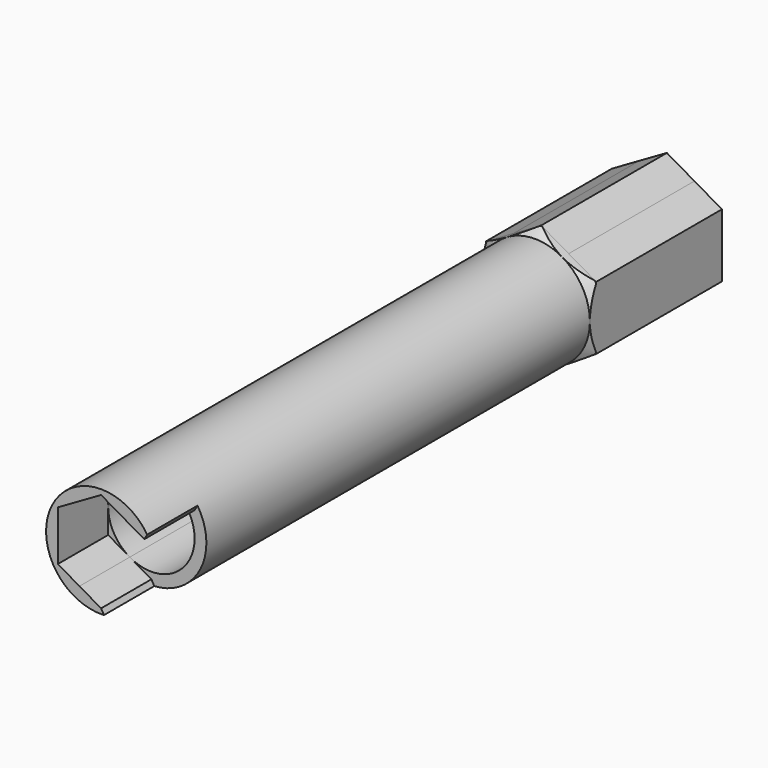
from build123d import *

# Parameters (mm, degrees)
F0_R         = 7
F1_DEPTH     = 70
F2_DEPTH     = 62
F3_R         = 5.5
F4_DEPTH     = 20
F6_DEPTH     = 8
F7_T4_ANGLE  = 59.9999999128
F7_T10_ANGLE = 59.9999996333
F7_T16_ANGLE = 60.0000004539
F7_T22_ANGLE = 59.9999999128
F7_T28_ANGLE = 60.0000002811
F7_T34_ANGLE = 59.9999998061


# Not quite as in the source:
# - a fillet or chamfer that OpenCascade refuses, or shapes differently, is made with other operations: its cross-section is extruded or revolved along the edge and cut away or added


with BuildPart() as f1:
    # F0 (on Front) → F1 (new body)
    with BuildSketch(Plane.XZ):
        Circle(F0_R)
        Polygon((2.7500007272, 4.7631393009), (5.5, 3.1754264805), (5.5, 0), (5.5, -3.1754264805), (2.7499994424, -4.7631400427), (0, -6.3508529611), (-2.7500008008, -4.7631392585), (-5.5, -3.1754264805), (-5.5, 0), (-5.5, 3.1754264805), (-2.7500002446, 4.7631395796), (0, 6.3508529611), align=None, mode=Mode.SUBTRACT)
    extrude(amount=F1_DEPTH)

    # F0 (on Front) → F2 (join)
    with BuildSketch(Plane.XZ):
        with BuildLine():
            Line((5.5, -3.1754264805), (5.5, 0))
            ThreePointArc((5.5, 0), (4.7631395599, -2.7500002788), (2.7499994424, -4.7631400427))
            Line((2.7499994424, -4.7631400427), (5.5, -3.1754264805))
        make_face()
        with BuildLine():
            Line((0, -6.3508529611), (2.7499994424, -4.7631400427))
            ThreePointArc((2.7499994424, -4.7631400427), (-7.842e-07, -5.5), (-2.7500008008, -4.7631392585))
            Line((-2.7500008008, -4.7631392585), (0, -6.3508529611))
        make_face()
        with BuildLine():
            Line((-5.5, -3.1754264805), (-2.7500008008, -4.7631392585))
            ThreePointArc((-2.7500008008, -4.7631392585), (-4.763139952, -2.7499995996), (-5.5, 0))
            Line((-5.5, 0), (-5.5, -3.1754264805))
        make_face()
        with BuildLine():
            ThreePointArc((-5.5, 0), (-4.7631397914, 2.7499998777), (-2.7500002446, 4.7631395796))
            Line((-2.7500002446, 4.7631395796), (-5.5, 3.1754264805))
            Line((-5.5, 3.1754264805), (-5.5, 0))
        make_face()
        with BuildLine():
            ThreePointArc((-2.7500002446, 4.7631395796), (2.787e-07, 5.5), (2.7500007272, 4.7631393009))
            Line((2.7500007272, 4.7631393009), (0, 6.3508529611))
            Line((0, 6.3508529611), (-2.7500002446, 4.7631395796))
        make_face()
        with BuildLine():
            Line((5.5, 0), (5.5, 3.1754264805))
            Line((5.5, 3.1754264805), (2.7500007272, 4.7631393009))
            ThreePointArc((2.7500007272, 4.7631393009), (4.7631399308, 2.7499996364), (5.5, 0))
        make_face()
    extrude(amount=F2_DEPTH)

    # F3 (on face) → F4 (join)
    with BuildSketch(Plane(origin=(0, 0, 0), x_dir=(-1, 0, 0), z_dir=(0, 1, 0))):
        with BuildLine():
            Line((-7, 0), (-7, -4.0414518843))
            Line((-7, -4.0414518843), (-3.5000000457, -6.0621778001))
            ThreePointArc((-3.5000000457, -6.0621778001), (-6.0621778397, -3.4999999772), (-7, 0))
        make_face()
        with BuildLine():
            Line((-7, 4.0414518843), (-7, 0))
            ThreePointArc((-7, 0), (-6.0621778147, 3.5000000204), (-3.4999999591, 6.0621778501))
            Line((-3.4999999591, 6.0621778501), (-7, 4.0414518843))
        make_face()
        with BuildLine():
            ThreePointArc((-3.4999999591, 6.0621778501), (-6.0621778147, 3.5000000204), (-7, 0))
            ThreePointArc((-7, 0), (-6.0621778397, -3.4999999772), (-3.5000000457, -6.0621778001))
            ThreePointArc((-3.5000000457, -6.0621778001), (-3.61e-08, -7), (3.4999999831, -6.0621778362))
            ThreePointArc((3.4999999831, -6.0621778362), (6.0621778216, -3.5000000084), (7, 0))
            ThreePointArc((7, 0), (6.06217782, 3.5000000113), (3.4999999774, 6.0621778395))
            ThreePointArc((3.4999999774, 6.0621778395), (1.05e-08, 7), (-3.4999999591, 6.0621778501))
        make_face()
        Circle(F3_R, mode=Mode.SUBTRACT)
        with BuildLine():
            ThreePointArc((3.4999999831, -6.0621778362), (-3.61e-08, -7), (-3.5000000457, -6.0621778001))
            Line((-3.5000000457, -6.0621778001), (0, -8.0829037687))
            Line((0, -8.0829037687), (3.4999999831, -6.0621778362))
        make_face()
        with BuildLine():
            Line((0, 8.0829037687), (-3.4999999591, 6.0621778501))
            ThreePointArc((-3.4999999591, 6.0621778501), (1.05e-08, 7), (3.4999999774, 6.0621778395))
            Line((3.4999999774, 6.0621778395), (0, 8.0829037687))
        make_face()
        with BuildLine():
            ThreePointArc((7, 0), (6.0621778216, -3.5000000084), (3.4999999831, -6.0621778362))
            Line((3.4999999831, -6.0621778362), (7, -4.0414518843))
            Line((7, -4.0414518843), (7, 0))
        make_face()
        with BuildLine():
            Line((7, 4.0414518843), (3.4999999774, 6.0621778395))
            ThreePointArc((3.4999999774, 6.0621778395), (6.06217782, 3.5000000113), (7, 0))
            Line((7, 0), (7, 4.0414518843))
        make_face()
    extrude(amount=F4_DEPTH)

    # F5 (on face) → F6 (cut, through all)
    with BuildSketch(Plane.XZ.offset(70)):
        with BuildLine():
            Line((5.5, 3.1754264805), (5.5, -3.1754264805))
            Line((5.5, -3.1754264805), (5.869161212, -3.814832456))
            ThreePointArc((5.869161212, -3.814832456), (6.7113384837, -1.9894561463), (7, 0))
            ThreePointArc((7, 0), (6.7113384837, 1.9894561463), (5.869161212, 3.814832456))
            Line((5.869161212, 3.814832456), (5.5, 3.1754264805))
        make_face()
        with BuildLine():
            Line((5.869161212, -3.814832456), (5.5, -3.1754264805))
            Line((5.5, -3.1754264805), (0, -6.3508529611))
            Line((0, -6.3508529611), (0.369161212, -6.9902589365))
            ThreePointArc((0.369161212, -6.9902589365), (3.5, -6.0621778265), (5.869161212, -3.814832456))
        make_face()
    extrude(amount=-F6_DEPTH, mode=Mode.SUBTRACT)

    # F7: chamfer of 1 on 6 edges, made by hand


with BuildPart() as f7_tool2:
    # F7_s3 → F7_t4 (revolve)
    with BuildSketch(Plane.XY):
        Polygon((-7, -1), (-8, 0), (-7, 0), align=None)
    revolve(axis=Axis((0, 0, 0), (0, -1, 0)), revolution_arc=F7_T4_ANGLE)

    split(bisect_by=Plane.YZ.offset(-7), keep=Keep.TOP)

    split(bisect_by=Plane(origin=(-3.5, 0, -6.0621778265), x_dir=(0, 1, 0), z_dir=(0.5, 0, 0.8660254038)), keep=Keep.TOP)


with BuildPart() as f1_1:
    add(f1.part)

    # F7_t1: union F7_tool2
    add(f7_tool2.part)


with BuildPart() as f7_tool8:
    # F7_s9 → F7_t10 (revolve)
    with BuildSketch(Plane.XY):
        Polygon((7, -1), (8, 0), (7, 0), align=None)
    revolve(axis=Axis((0, 0, 0), (0, -1, 0)), revolution_arc=F7_T10_ANGLE)

    split(bisect_by=Plane(origin=(3.5, 0, 6.0621778265), x_dir=(0, 1, 0), z_dir=(-0.5, 0, -0.8660254038)), keep=Keep.TOP)

    split(bisect_by=Plane.YZ.offset(7), keep=Keep.BOTTOM)


with BuildPart() as f1_2:
    add(f1_1.part)

    # F7_t7: union F7_tool8
    add(f7_tool8.part)


with BuildPart() as f7_tool14:
    # F7_s15 → F7_t16 (revolve)
    with BuildSketch(Plane(origin=(0, 0, 0), x_dir=(0, 1, 0), z_dir=(0.8660254006, 0, -0.5000000055))):
        Polygon((-1, 7), (0, 8), (0, 7), align=None)
    revolve(axis=Axis((0, 0, 0), (0, -1, 0)), revolution_arc=F7_T16_ANGLE)

    split(bisect_by=Plane(origin=(3.5, 0, 6.0621778265), x_dir=(0, 1, 0), z_dir=(-0.5, 0, -0.8660254038)), keep=Keep.TOP)

    split(bisect_by=Plane(origin=(-3.5, 0, 6.0621778265), x_dir=(0, 1, 0), z_dir=(0.5, 0, -0.8660254038)), keep=Keep.TOP)


with BuildPart() as f1_3:
    add(f1_2.part)

    # F7_t13: union F7_tool14
    add(f7_tool14.part)


with BuildPart() as f7_tool20:
    # F7_s21 → F7_t22 (revolve)
    with BuildSketch(Plane(origin=(0, 0, 0), x_dir=(0, 1, 0), z_dir=(0.866025403, 0, 0.5000000013))):
        Polygon((-1, 7), (0, 8), (0, 7), align=None)
    revolve(axis=Axis((0, 0, 0), (0, -1, 0)), revolution_arc=F7_T22_ANGLE)

    split(bisect_by=Plane(origin=(-3.5, 0, 6.0621778265), x_dir=(0, 1, 0), z_dir=(0.5, 0, -0.8660254038)), keep=Keep.TOP)

    split(bisect_by=Plane.YZ.offset(-7), keep=Keep.TOP)


with BuildPart() as f1_4:
    add(f1_3.part)

    # F7_t19: union F7_tool20
    add(f7_tool20.part)


with BuildPart() as f7_tool26:
    # F7_s27 → F7_t28 (revolve)
    with BuildSketch(Plane(origin=(0, 0, 0), x_dir=(0, 1, 0), z_dir=(-0.866025403, 0, 0.5000000013))):
        Polygon((-1, 7), (0, 8), (0, 7), align=None)
    revolve(axis=Axis((0, 0, 0), (0, -1, 0)), revolution_arc=F7_T28_ANGLE)

    split(bisect_by=Plane(origin=(3.5, 0, -6.0621778265), x_dir=(0, 1, 0), z_dir=(-0.5, 0, 0.8660254038)), keep=Keep.TOP)

    split(bisect_by=Plane(origin=(-3.5, 0, -6.0621778265), x_dir=(0, 1, 0), z_dir=(0.5, 0, 0.8660254038)), keep=Keep.TOP)


with BuildPart() as f1_5:
    add(f1_4.part)

    # F7_t25: union F7_tool26
    add(f7_tool26.part)


with BuildPart() as f7_tool32:
    # F7_s33 → F7_t34 (revolve)
    with BuildSketch(Plane(origin=(0, 0, 0), x_dir=(0, 1, 0), z_dir=(-0.8660254021, 0, -0.5000000029))):
        Polygon((-1, 7), (0, 8), (0, 7), align=None)
    revolve(axis=Axis((0, 0, 0), (0, -1, 0)), revolution_arc=F7_T34_ANGLE)

    split(bisect_by=Plane(origin=(3.5, 0, -6.0621778265), x_dir=(0, 1, 0), z_dir=(-0.5, 0, 0.8660254038)), keep=Keep.TOP)

    split(bisect_by=Plane.YZ.offset(7), keep=Keep.BOTTOM)


with BuildPart() as f1_6:
    add(f1_5.part)

    # F7_t31: union F7_tool32
    add(f7_tool32.part)


solid = f1_6.part
